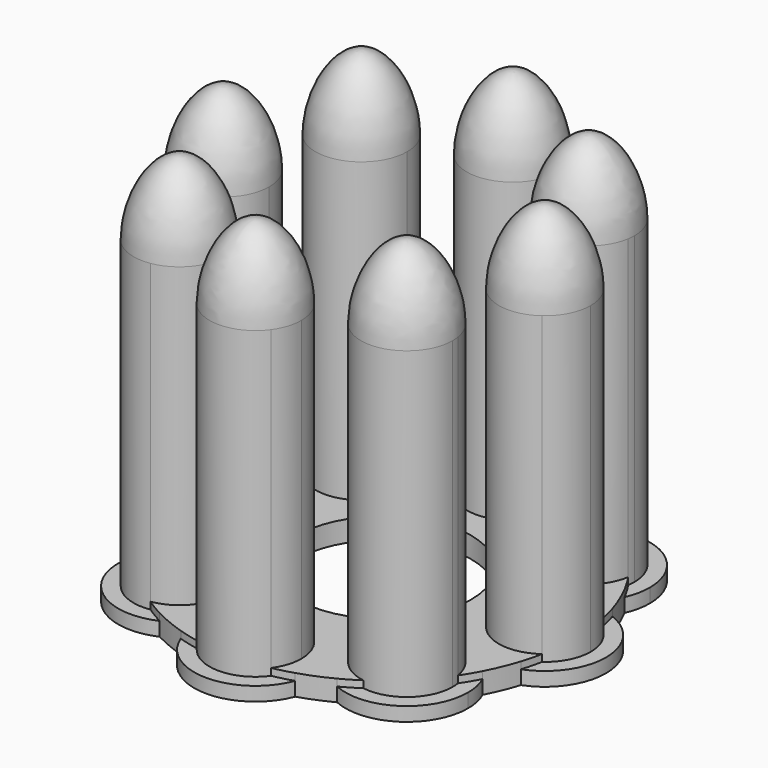
from build123d import *

# Parameters (mm, degrees)
F0_R            = 7.9375
F1_DEPTH        = 0.635
F2_DEPTH        = 1.27
F3_DEPTH        = 27.813
F5_COPIES_COUNT = 8


# Not quite as in the source:
# - a pattern or mirror of a feature is missing from the dataset's text; its kind, count and spacing are read off the source's solid


with BuildPart() as f1:
    # F0 (on Top) → F1 (new body)
    with BuildSketch(Plane.XY):
        with BuildLine():
            ThreePointArc((-5.219470135, 16.6642142857), (-1.0147277679, 9.1734047727), (5.588, 14.6685))
            ThreePointArc((5.588, 14.6685), (5.4950952273, 15.6832277679), (5.219470135, 16.6642142857))
            ThreePointArc((5.219470135, 16.6642142857), (4.3120566918, 16.9217337568), (3.3920620288, 17.1298809524))
            ThreePointArc((3.3920620288, 17.1298809524), (3.986264728, 15.96239896), (4.191, 14.6685))
            ThreePointArc((4.191, 14.6685), (-1.29389896, 10.682235272), (-3.3920620288, 17.1298809524))
            ThreePointArc((-3.3920620288, 17.1298809524), (-4.3120566918, 16.9217337568), (-5.219470135, 16.6642142857))
        make_face()
        with BuildLine():
            ThreePointArc((9.7141049196, 14.5112050451), (8.9163881613, 15.0145572165), (8.0926561979, 15.4741016512))
            ThreePointArc((8.0926561979, 15.4741016512), (6.4208831266, 6.4208831266), (15.4741016512, 8.0926561979))
            ThreePointArc((15.4741016512, 8.0926561979), (15.0145572165, 8.9163881613), (14.5112050451, 9.7141049196))
            ThreePointArc((14.5112050451, 9.7141049196), (7.4087112999, 7.4087112999), (9.7141049196, 14.5112050451))
        make_face()
        with BuildLine():
            ThreePointArc((17.1298809524, 3.3920620288), (16.9217337568, 4.3120566918), (16.6642142857, 5.219470135))
            ThreePointArc((16.6642142857, 5.219470135), (9.0805, 0), (16.6642142857, -5.219470135))
            ThreePointArc((16.6642142857, -5.219470135), (16.9217337568, -4.3120566918), (17.1298809524, -3.3920620288))
            ThreePointArc((17.1298809524, -3.3920620288), (10.4775, 0), (17.1298809524, 3.3920620288))
        make_face()
        with BuildLine():
            ThreePointArc((14.5112050451, -9.7141049196), (15.0145572165, -8.9163881613), (15.4741016512, -8.0926561979))
            ThreePointArc((15.4741016512, -8.0926561979), (6.4208831266, -6.4208831266), (8.0926561979, -15.4741016512))
            ThreePointArc((8.0926561979, -15.4741016512), (8.9163881613, -15.0145572165), (9.7141049196, -14.5112050451))
            ThreePointArc((9.7141049196, -14.5112050451), (7.4087112999, -7.4087112999), (14.5112050451, -9.7141049196))
        make_face()
        with BuildLine():
            ThreePointArc((3.3920620288, -17.1298809524), (4.3120566918, -16.9217337568), (5.219470135, -16.6642142857))
            ThreePointArc((5.219470135, -16.6642142857), (5.4950952273, -15.6832277679), (5.588, -14.6685))
            ThreePointArc((5.588, -14.6685), (-1.0147277679, -9.1734047727), (-5.219470135, -16.6642142857))
            ThreePointArc((-5.219470135, -16.6642142857), (-4.3120566918, -16.9217337568), (-3.3920620288, -17.1298809524))
            ThreePointArc((-3.3920620288, -17.1298809524), (-1.29389896, -10.682235272), (4.191, -14.6685))
            ThreePointArc((4.191, -14.6685), (3.986264728, -15.96239896), (3.3920620288, -17.1298809524))
        make_face()
        with BuildLine():
            ThreePointArc((-4.7841958198, -10.3721958198), (-9.2068001329, -4.907070305), (-15.4741016512, -8.0926561979))
            ThreePointArc((-15.4741016512, -8.0926561979), (-15.0145572165, -8.9163881613), (-14.5112050451, -9.7141049196))
            ThreePointArc((-14.5112050451, -9.7141049196), (-10.0421251177, -6.1942137314), (-6.1811958198, -10.3721958198))
            ThreePointArc((-6.1811958198, -10.3721958198), (-7.1845211216, -13.0930800545), (-9.7141049196, -14.5112050451))
            ThreePointArc((-9.7141049196, -14.5112050451), (-8.9163881613, -15.0145572165), (-8.0926561979, -15.4741016512))
            ThreePointArc((-8.0926561979, -15.4741016512), (-5.6837093153, -13.4125639384), (-4.7841958198, -10.3721958198))
        make_face()
        with BuildLine():
            ThreePointArc((-9.0805, 0), (-11.5004017872, 4.6031399842), (-16.6642142857, 5.219470135))
            ThreePointArc((-16.6642142857, 5.219470135), (-16.9217337568, 4.3120566918), (-17.1298809524, 3.3920620288))
            ThreePointArc((-17.1298809524, 3.3920620288), (-12.764709908, 3.7336395495), (-10.4775, 0))
            ThreePointArc((-10.4775, 0), (-12.764709908, -3.7336395495), (-17.1298809524, -3.3920620288))
            ThreePointArc((-17.1298809524, -3.3920620288), (-16.9217337568, -4.3120566918), (-16.6642142857, -5.219470135))
            ThreePointArc((-16.6642142857, -5.219470135), (-11.5004017872, -4.6031399842), (-9.0805, 0))
        make_face()
        with BuildLine():
            ThreePointArc((-4.7841958198, 10.3721958198), (-5.6837093153, 13.4125639384), (-8.0926561979, 15.4741016512))
            ThreePointArc((-8.0926561979, 15.4741016512), (-8.9163881613, 15.0145572165), (-9.7141049196, 14.5112050451))
            ThreePointArc((-9.7141049196, 14.5112050451), (-7.1845211216, 13.0930800545), (-6.1811958198, 10.3721958198))
            ThreePointArc((-6.1811958198, 10.3721958198), (-10.0421251177, 6.1942137314), (-14.5112050451, 9.7141049196))
            ThreePointArc((-14.5112050451, 9.7141049196), (-15.0145572165, 8.9163881613), (-15.4741016512, 8.0926561979))
            ThreePointArc((-15.4741016512, 8.0926561979), (-9.2068001329, 4.907070305), (-4.7841958198, 10.3721958198))
        make_face()
        with BuildLine():
            ThreePointArc((5.219470135, 16.6642142857), (5.4950952273, 15.6832277679), (5.588, 14.6685))
            ThreePointArc((5.588, 14.6685), (-1.0147277679, 9.1734047727), (-5.219470135, 16.6642142857))
            ThreePointArc((-5.219470135, 16.6642142857), (-6.6826094377, 16.1332463365), (-8.0926561979, 15.4741016512))
            ThreePointArc((-8.0926561979, 15.4741016512), (-5.6837093153, 13.4125639384), (-4.7841958198, 10.3721958198))
            ThreePointArc((-4.7841958198, 10.3721958198), (-9.2068001329, 4.907070305), (-15.4741016512, 8.0926561979))
            ThreePointArc((-15.4741016512, 8.0926561979), (-16.1332463365, 6.6826094377), (-16.6642142857, 5.219470135))
            ThreePointArc((-16.6642142857, 5.219470135), (-11.5004017872, 4.6031399842), (-9.0805, 0))
            ThreePointArc((-9.0805, 0), (-11.5004017872, -4.6031399842), (-16.6642142857, -5.219470135))
            ThreePointArc((-16.6642142857, -5.219470135), (-16.1332463365, -6.6826094377), (-15.4741016512, -8.0926561979))
            ThreePointArc((-15.4741016512, -8.0926561979), (-9.2068001329, -4.907070305), (-4.7841958198, -10.3721958198))
            ThreePointArc((-4.7841958198, -10.3721958198), (-5.6837093153, -13.4125639384), (-8.0926561979, -15.4741016512))
            ThreePointArc((-8.0926561979, -15.4741016512), (-6.6826094377, -16.1332463365), (-5.219470135, -16.6642142857))
            ThreePointArc((-5.219470135, -16.6642142857), (-1.0147277679, -9.1734047727), (5.588, -14.6685))
            ThreePointArc((5.588, -14.6685), (5.4950952273, -15.6832277679), (5.219470135, -16.6642142857))
            ThreePointArc((5.219470135, -16.6642142857), (6.6826094377, -16.1332463365), (8.0926561979, -15.4741016512))
            ThreePointArc((8.0926561979, -15.4741016512), (6.4208831266, -6.4208831266), (15.4741016512, -8.0926561979))
            ThreePointArc((15.4741016512, -8.0926561979), (16.1332463365, -6.6826094377), (16.6642142857, -5.219470135))
            ThreePointArc((16.6642142857, -5.219470135), (9.0805, 0), (16.6642142857, 5.219470135))
            ThreePointArc((16.6642142857, 5.219470135), (16.1332463365, 6.6826094377), (15.4741016512, 8.0926561979))
            ThreePointArc((15.4741016512, 8.0926561979), (6.4208831266, 6.4208831266), (8.0926561979, 15.4741016512))
            ThreePointArc((8.0926561979, 15.4741016512), (6.6826094377, 16.1332463365), (5.219470135, 16.6642142857))
        make_face()
        Circle(F0_R, mode=Mode.SUBTRACT)
    extrude(amount=F1_DEPTH)

    # F0 (on Top) → F2 (join)
    with BuildSketch(Plane.XY):
        with BuildLine():
            ThreePointArc((-5.219470135, 16.6642142857), (-1.0147277679, 9.1734047727), (5.588, 14.6685))
            ThreePointArc((5.588, 14.6685), (5.4950952273, 15.6832277679), (5.219470135, 16.6642142857))
            ThreePointArc((5.219470135, 16.6642142857), (4.3120566918, 16.9217337568), (3.3920620288, 17.1298809524))
            ThreePointArc((3.3920620288, 17.1298809524), (3.986264728, 15.96239896), (4.191, 14.6685))
            ThreePointArc((4.191, 14.6685), (-1.29389896, 10.682235272), (-3.3920620288, 17.1298809524))
            ThreePointArc((-3.3920620288, 17.1298809524), (-4.3120566918, 16.9217337568), (-5.219470135, 16.6642142857))
        make_face()
        with BuildLine():
            ThreePointArc((5.219470135, 16.6642142857), (5.4950952273, 15.6832277679), (5.588, 14.6685))
            ThreePointArc((5.588, 14.6685), (-1.0147277679, 9.1734047727), (-5.219470135, 16.6642142857))
            ThreePointArc((-5.219470135, 16.6642142857), (-6.6826094377, 16.1332463365), (-8.0926561979, 15.4741016512))
            ThreePointArc((-8.0926561979, 15.4741016512), (-5.6837093153, 13.4125639384), (-4.7841958198, 10.3721958198))
            ThreePointArc((-4.7841958198, 10.3721958198), (-9.2068001329, 4.907070305), (-15.4741016512, 8.0926561979))
            ThreePointArc((-15.4741016512, 8.0926561979), (-16.1332463365, 6.6826094377), (-16.6642142857, 5.219470135))
            ThreePointArc((-16.6642142857, 5.219470135), (-11.5004017872, 4.6031399842), (-9.0805, 0))
            ThreePointArc((-9.0805, 0), (-11.5004017872, -4.6031399842), (-16.6642142857, -5.219470135))
            ThreePointArc((-16.6642142857, -5.219470135), (-16.1332463365, -6.6826094377), (-15.4741016512, -8.0926561979))
            ThreePointArc((-15.4741016512, -8.0926561979), (-9.2068001329, -4.907070305), (-4.7841958198, -10.3721958198))
            ThreePointArc((-4.7841958198, -10.3721958198), (-5.6837093153, -13.4125639384), (-8.0926561979, -15.4741016512))
            ThreePointArc((-8.0926561979, -15.4741016512), (-6.6826094377, -16.1332463365), (-5.219470135, -16.6642142857))
            ThreePointArc((-5.219470135, -16.6642142857), (-1.0147277679, -9.1734047727), (5.588, -14.6685))
            ThreePointArc((5.588, -14.6685), (5.4950952273, -15.6832277679), (5.219470135, -16.6642142857))
            ThreePointArc((5.219470135, -16.6642142857), (6.6826094377, -16.1332463365), (8.0926561979, -15.4741016512))
            ThreePointArc((8.0926561979, -15.4741016512), (6.4208831266, -6.4208831266), (15.4741016512, -8.0926561979))
            ThreePointArc((15.4741016512, -8.0926561979), (16.1332463365, -6.6826094377), (16.6642142857, -5.219470135))
            ThreePointArc((16.6642142857, -5.219470135), (9.0805, 0), (16.6642142857, 5.219470135))
            ThreePointArc((16.6642142857, 5.219470135), (16.1332463365, 6.6826094377), (15.4741016512, 8.0926561979))
            ThreePointArc((15.4741016512, 8.0926561979), (6.4208831266, 6.4208831266), (8.0926561979, 15.4741016512))
            ThreePointArc((8.0926561979, 15.4741016512), (6.6826094377, 16.1332463365), (5.219470135, 16.6642142857))
        make_face()
        Circle(F0_R, mode=Mode.SUBTRACT)
        with BuildLine():
            ThreePointArc((3.3920620288, 17.1298809524), (4.3120566918, 16.9217337568), (5.219470135, 16.6642142857))
            ThreePointArc((5.219470135, 16.6642142857), (0, 20.2565), (-5.219470135, 16.6642142857))
            ThreePointArc((-5.219470135, 16.6642142857), (-4.3120566918, 16.9217337568), (-3.3920620288, 17.1298809524))
            ThreePointArc((-3.3920620288, 17.1298809524), (0, 18.8595), (3.3920620288, 17.1298809524))
        make_face()
        with BuildLine():
            ThreePointArc((15.9601958198, 10.3721958198), (13.4125639384, 15.0606823244), (8.0926561979, 15.4741016512))
            ThreePointArc((8.0926561979, 15.4741016512), (8.9163881613, 15.0145572165), (9.7141049196, 14.5112050451))
            ThreePointArc((9.7141049196, 14.5112050451), (13.0930800545, 13.559870518), (14.5631958198, 10.3721958198))
            ThreePointArc((14.5631958198, 10.3721958198), (14.5501779083, 10.0421251177), (14.5112050451, 9.7141049196))
            ThreePointArc((14.5112050451, 9.7141049196), (15.0145572165, 8.9163881613), (15.4741016512, 8.0926561979))
            ThreePointArc((15.4741016512, 8.0926561979), (15.8373213347, 9.2068001329), (15.9601958198, 10.3721958198))
        make_face()
        with BuildLine():
            ThreePointArc((9.7141049196, 14.5112050451), (8.9163881613, 15.0145572165), (8.0926561979, 15.4741016512))
            ThreePointArc((8.0926561979, 15.4741016512), (6.4208831266, 6.4208831266), (15.4741016512, 8.0926561979))
            ThreePointArc((15.4741016512, 8.0926561979), (15.0145572165, 8.9163881613), (14.5112050451, 9.7141049196))
            ThreePointArc((14.5112050451, 9.7141049196), (7.4087112999, 7.4087112999), (9.7141049196, 14.5112050451))
        make_face()
        with BuildLine():
            ThreePointArc((-4.7841958198, 10.3721958198), (-5.6837093153, 13.4125639384), (-8.0926561979, 15.4741016512))
            ThreePointArc((-8.0926561979, 15.4741016512), (-8.9163881613, 15.0145572165), (-9.7141049196, 14.5112050451))
            ThreePointArc((-9.7141049196, 14.5112050451), (-7.1845211216, 13.0930800545), (-6.1811958198, 10.3721958198))
            ThreePointArc((-6.1811958198, 10.3721958198), (-10.0421251177, 6.1942137314), (-14.5112050451, 9.7141049196))
            ThreePointArc((-14.5112050451, 9.7141049196), (-15.0145572165, 8.9163881613), (-15.4741016512, 8.0926561979))
            ThreePointArc((-15.4741016512, 8.0926561979), (-9.2068001329, 4.907070305), (-4.7841958198, 10.3721958198))
        make_face()
        with BuildLine():
            ThreePointArc((-9.7141049196, 14.5112050451), (-8.9163881613, 15.0145572165), (-8.0926561979, 15.4741016512))
            ThreePointArc((-8.0926561979, 15.4741016512), (-14.3235085131, 14.3235085131), (-15.4741016512, 8.0926561979))
            ThreePointArc((-15.4741016512, 8.0926561979), (-15.0145572165, 8.9163881613), (-14.5112050451, 9.7141049196))
            ThreePointArc((-14.5112050451, 9.7141049196), (-13.3356803398, 13.3356803398), (-9.7141049196, 14.5112050451))
        make_face()
        with BuildLine():
            ThreePointArc((20.2565, 0), (19.2716399842, 3.1680982128), (16.6642142857, 5.219470135))
            ThreePointArc((16.6642142857, 5.219470135), (16.9217337568, 4.3120566918), (17.1298809524, 3.3920620288))
            ThreePointArc((17.1298809524, 3.3920620288), (18.4021395495, 1.903790092), (18.8595, 0))
            ThreePointArc((18.8595, 0), (18.4021395495, -1.903790092), (17.1298809524, -3.3920620288))
            ThreePointArc((17.1298809524, -3.3920620288), (16.9217337568, -4.3120566918), (16.6642142857, -5.219470135))
            ThreePointArc((16.6642142857, -5.219470135), (19.2716399842, -3.1680982128), (20.2565, 0))
        make_face()
        with BuildLine():
            ThreePointArc((17.1298809524, 3.3920620288), (16.9217337568, 4.3120566918), (16.6642142857, 5.219470135))
            ThreePointArc((16.6642142857, 5.219470135), (9.0805, 0), (16.6642142857, -5.219470135))
            ThreePointArc((16.6642142857, -5.219470135), (16.9217337568, -4.3120566918), (17.1298809524, -3.3920620288))
            ThreePointArc((17.1298809524, -3.3920620288), (10.4775, 0), (17.1298809524, 3.3920620288))
        make_face()
        with BuildLine():
            ThreePointArc((-9.0805, 0), (-11.5004017872, 4.6031399842), (-16.6642142857, 5.219470135))
            ThreePointArc((-16.6642142857, 5.219470135), (-16.9217337568, 4.3120566918), (-17.1298809524, 3.3920620288))
            ThreePointArc((-17.1298809524, 3.3920620288), (-12.764709908, 3.7336395495), (-10.4775, 0))
            ThreePointArc((-10.4775, 0), (-12.764709908, -3.7336395495), (-17.1298809524, -3.3920620288))
            ThreePointArc((-17.1298809524, -3.3920620288), (-16.9217337568, -4.3120566918), (-16.6642142857, -5.219470135))
            ThreePointArc((-16.6642142857, -5.219470135), (-11.5004017872, -4.6031399842), (-9.0805, 0))
        make_face()
        with BuildLine():
            ThreePointArc((-17.1298809524, 3.3920620288), (-16.9217337568, 4.3120566918), (-16.6642142857, 5.219470135))
            ThreePointArc((-16.6642142857, 5.219470135), (-20.2565, 0), (-16.6642142857, -5.219470135))
            ThreePointArc((-16.6642142857, -5.219470135), (-16.9217337568, -4.3120566918), (-17.1298809524, -3.3920620288))
            ThreePointArc((-17.1298809524, -3.3920620288), (-18.8595, 0), (-17.1298809524, 3.3920620288))
        make_face()
        with BuildLine():
            ThreePointArc((15.9601958198, -10.3721958198), (15.8373213347, -9.2068001329), (15.4741016512, -8.0926561979))
            ThreePointArc((15.4741016512, -8.0926561979), (15.0145572165, -8.9163881613), (14.5112050451, -9.7141049196))
            ThreePointArc((14.5112050451, -9.7141049196), (14.5501779083, -10.0421251177), (14.5631958198, -10.3721958198))
            ThreePointArc((14.5631958198, -10.3721958198), (13.0930800545, -13.559870518), (9.7141049196, -14.5112050451))
            ThreePointArc((9.7141049196, -14.5112050451), (8.9163881613, -15.0145572165), (8.0926561979, -15.4741016512))
            ThreePointArc((8.0926561979, -15.4741016512), (13.4125639384, -15.0606823244), (15.9601958198, -10.3721958198))
        make_face()
        with BuildLine():
            ThreePointArc((14.5112050451, -9.7141049196), (15.0145572165, -8.9163881613), (15.4741016512, -8.0926561979))
            ThreePointArc((15.4741016512, -8.0926561979), (6.4208831266, -6.4208831266), (8.0926561979, -15.4741016512))
            ThreePointArc((8.0926561979, -15.4741016512), (8.9163881613, -15.0145572165), (9.7141049196, -14.5112050451))
            ThreePointArc((9.7141049196, -14.5112050451), (7.4087112999, -7.4087112999), (14.5112050451, -9.7141049196))
        make_face()
        with BuildLine():
            ThreePointArc((-4.7841958198, -10.3721958198), (-9.2068001329, -4.907070305), (-15.4741016512, -8.0926561979))
            ThreePointArc((-15.4741016512, -8.0926561979), (-15.0145572165, -8.9163881613), (-14.5112050451, -9.7141049196))
            ThreePointArc((-14.5112050451, -9.7141049196), (-10.0421251177, -6.1942137314), (-6.1811958198, -10.3721958198))
            ThreePointArc((-6.1811958198, -10.3721958198), (-7.1845211216, -13.0930800545), (-9.7141049196, -14.5112050451))
            ThreePointArc((-9.7141049196, -14.5112050451), (-8.9163881613, -15.0145572165), (-8.0926561979, -15.4741016512))
            ThreePointArc((-8.0926561979, -15.4741016512), (-5.6837093153, -13.4125639384), (-4.7841958198, -10.3721958198))
        make_face()
        with BuildLine():
            ThreePointArc((-14.5112050451, -9.7141049196), (-15.0145572165, -8.9163881613), (-15.4741016512, -8.0926561979))
            ThreePointArc((-15.4741016512, -8.0926561979), (-14.3235085131, -14.3235085131), (-8.0926561979, -15.4741016512))
            ThreePointArc((-8.0926561979, -15.4741016512), (-8.9163881613, -15.0145572165), (-9.7141049196, -14.5112050451))
            ThreePointArc((-9.7141049196, -14.5112050451), (-13.3356803398, -13.3356803398), (-14.5112050451, -9.7141049196))
        make_face()
        with BuildLine():
            ThreePointArc((-5.219470135, -16.6642142857), (0, -20.2565), (5.219470135, -16.6642142857))
            ThreePointArc((5.219470135, -16.6642142857), (4.3120566918, -16.9217337568), (3.3920620288, -17.1298809524))
            ThreePointArc((3.3920620288, -17.1298809524), (0, -18.8595), (-3.3920620288, -17.1298809524))
            ThreePointArc((-3.3920620288, -17.1298809524), (-4.3120566918, -16.9217337568), (-5.219470135, -16.6642142857))
        make_face()
        with BuildLine():
            ThreePointArc((3.3920620288, -17.1298809524), (4.3120566918, -16.9217337568), (5.219470135, -16.6642142857))
            ThreePointArc((5.219470135, -16.6642142857), (5.4950952273, -15.6832277679), (5.588, -14.6685))
            ThreePointArc((5.588, -14.6685), (-1.0147277679, -9.1734047727), (-5.219470135, -16.6642142857))
            ThreePointArc((-5.219470135, -16.6642142857), (-4.3120566918, -16.9217337568), (-3.3920620288, -17.1298809524))
            ThreePointArc((-3.3920620288, -17.1298809524), (-1.29389896, -10.682235272), (4.191, -14.6685))
            ThreePointArc((4.191, -14.6685), (3.986264728, -15.96239896), (3.3920620288, -17.1298809524))
        make_face()
        with BuildLine():
            ThreePointArc((-3.3920620288, -17.1298809524), (0, -18.8595), (3.3920620288, -17.1298809524))
            ThreePointArc((3.3920620288, -17.1298809524), (0, -17.4625), (-3.3920620288, -17.1298809524))
        make_face()
        with BuildLine():
            ThreePointArc((-3.3920620288, -17.1298809524), (0, -17.4625), (3.3920620288, -17.1298809524))
            ThreePointArc((3.3920620288, -17.1298809524), (3.986264728, -15.96239896), (4.191, -14.6685))
            ThreePointArc((4.191, -14.6685), (-1.29389896, -10.682235272), (-3.3920620288, -17.1298809524))
        make_face()
        with BuildLine():
            ThreePointArc((9.7141049196, -14.5112050451), (12.3478521665, -12.3478521665), (14.5112050451, -9.7141049196))
            ThreePointArc((14.5112050451, -9.7141049196), (7.4087112999, -7.4087112999), (9.7141049196, -14.5112050451))
        make_face()
        with BuildLine():
            ThreePointArc((14.5631958198, -10.3721958198), (14.5501779083, -10.0421251177), (14.5112050451, -9.7141049196))
            ThreePointArc((14.5112050451, -9.7141049196), (12.3478521665, -12.3478521665), (9.7141049196, -14.5112050451))
            ThreePointArc((9.7141049196, -14.5112050451), (13.0930800545, -13.559870518), (14.5631958198, -10.3721958198))
        make_face()
        with BuildLine():
            ThreePointArc((18.8595, 0), (18.4021395495, 1.903790092), (17.1298809524, 3.3920620288))
            ThreePointArc((17.1298809524, 3.3920620288), (17.3791463021, 1.7041655024), (17.4625, 0))
            ThreePointArc((17.4625, 0), (17.3791463021, -1.7041655024), (17.1298809524, -3.3920620288))
            ThreePointArc((17.1298809524, -3.3920620288), (18.4021395495, -1.903790092), (18.8595, 0))
        make_face()
        with BuildLine():
            ThreePointArc((17.4625, 0), (17.3791463021, 1.7041655024), (17.1298809524, 3.3920620288))
            ThreePointArc((17.1298809524, 3.3920620288), (10.4775, 0), (17.1298809524, -3.3920620288))
            ThreePointArc((17.1298809524, -3.3920620288), (17.3791463021, -1.7041655024), (17.4625, 0))
        make_face()
        with BuildLine():
            ThreePointArc((14.5112050451, 9.7141049196), (12.3478521665, 12.3478521665), (9.7141049196, 14.5112050451))
            ThreePointArc((9.7141049196, 14.5112050451), (7.4087112999, 7.4087112999), (14.5112050451, 9.7141049196))
        make_face()
        with BuildLine():
            ThreePointArc((14.5631958198, 10.3721958198), (13.0930800545, 13.559870518), (9.7141049196, 14.5112050451))
            ThreePointArc((9.7141049196, 14.5112050451), (12.3478521665, 12.3478521665), (14.5112050451, 9.7141049196))
            ThreePointArc((14.5112050451, 9.7141049196), (14.5501779083, 10.0421251177), (14.5631958198, 10.3721958198))
        make_face()
        with BuildLine():
            ThreePointArc((-6.1811958198, 10.3721958198), (-7.1845211216, 13.0930800545), (-9.7141049196, 14.5112050451))
            ThreePointArc((-9.7141049196, 14.5112050451), (-12.3478521665, 12.3478521665), (-14.5112050451, 9.7141049196))
            ThreePointArc((-14.5112050451, 9.7141049196), (-10.0421251177, 6.1942137314), (-6.1811958198, 10.3721958198))
        make_face()
        with BuildLine():
            ThreePointArc((-14.5112050451, 9.7141049196), (-12.3478521665, 12.3478521665), (-9.7141049196, 14.5112050451))
            ThreePointArc((-9.7141049196, 14.5112050451), (-13.3356803398, 13.3356803398), (-14.5112050451, 9.7141049196))
        make_face()
        with BuildLine():
            ThreePointArc((-10.4775, 0), (-12.764709908, 3.7336395495), (-17.1298809524, 3.3920620288))
            ThreePointArc((-17.1298809524, 3.3920620288), (-17.4625, 0), (-17.1298809524, -3.3920620288))
            ThreePointArc((-17.1298809524, -3.3920620288), (-12.764709908, -3.7336395495), (-10.4775, 0))
        make_face()
        with BuildLine():
            ThreePointArc((4.191, 14.6685), (3.986264728, 15.96239896), (3.3920620288, 17.1298809524))
            ThreePointArc((3.3920620288, 17.1298809524), (0, 17.4625), (-3.3920620288, 17.1298809524))
            ThreePointArc((-3.3920620288, 17.1298809524), (-1.29389896, 10.682235272), (4.191, 14.6685))
        make_face()
        with BuildLine():
            ThreePointArc((-3.3920620288, 17.1298809524), (0, 17.4625), (3.3920620288, 17.1298809524))
            ThreePointArc((3.3920620288, 17.1298809524), (0, 18.8595), (-3.3920620288, 17.1298809524))
        make_face()
        with BuildLine():
            ThreePointArc((-9.7141049196, -14.5112050451), (-12.3478521665, -12.3478521665), (-14.5112050451, -9.7141049196))
            ThreePointArc((-14.5112050451, -9.7141049196), (-13.3356803398, -13.3356803398), (-9.7141049196, -14.5112050451))
        make_face()
        with BuildLine():
            ThreePointArc((-6.1811958198, -10.3721958198), (-10.0421251177, -6.1942137314), (-14.5112050451, -9.7141049196))
            ThreePointArc((-14.5112050451, -9.7141049196), (-12.3478521665, -12.3478521665), (-9.7141049196, -14.5112050451))
            ThreePointArc((-9.7141049196, -14.5112050451), (-7.1845211216, -13.0930800545), (-6.1811958198, -10.3721958198))
        make_face()
        with BuildLine():
            ThreePointArc((-17.1298809524, -3.3920620288), (-17.4625, 0), (-17.1298809524, 3.3920620288))
            ThreePointArc((-17.1298809524, 3.3920620288), (-18.8595, 0), (-17.1298809524, -3.3920620288))
        make_face()
    extrude(amount=-F2_DEPTH)

    # F0 (on Top) → F3 (join)
    with BuildSketch(Plane.XY):
        with BuildLine():
            ThreePointArc((9.7141049196, -14.5112050451), (12.3478521665, -12.3478521665), (14.5112050451, -9.7141049196))
            ThreePointArc((14.5112050451, -9.7141049196), (7.4087112999, -7.4087112999), (9.7141049196, -14.5112050451))
        make_face()
        with BuildLine():
            ThreePointArc((14.5631958198, -10.3721958198), (14.5501779083, -10.0421251177), (14.5112050451, -9.7141049196))
            ThreePointArc((14.5112050451, -9.7141049196), (12.3478521665, -12.3478521665), (9.7141049196, -14.5112050451))
            ThreePointArc((9.7141049196, -14.5112050451), (13.0930800545, -13.559870518), (14.5631958198, -10.3721958198))
        make_face()
        with BuildLine():
            ThreePointArc((-3.3920620288, -17.1298809524), (0, -18.8595), (3.3920620288, -17.1298809524))
            ThreePointArc((3.3920620288, -17.1298809524), (0, -17.4625), (-3.3920620288, -17.1298809524))
        make_face()
        with BuildLine():
            ThreePointArc((-3.3920620288, -17.1298809524), (0, -17.4625), (3.3920620288, -17.1298809524))
            ThreePointArc((3.3920620288, -17.1298809524), (3.986264728, -15.96239896), (4.191, -14.6685))
            ThreePointArc((4.191, -14.6685), (-1.29389896, -10.682235272), (-3.3920620288, -17.1298809524))
        make_face()
        with BuildLine():
            ThreePointArc((-6.1811958198, -10.3721958198), (-10.0421251177, -6.1942137314), (-14.5112050451, -9.7141049196))
            ThreePointArc((-14.5112050451, -9.7141049196), (-12.3478521665, -12.3478521665), (-9.7141049196, -14.5112050451))
            ThreePointArc((-9.7141049196, -14.5112050451), (-7.1845211216, -13.0930800545), (-6.1811958198, -10.3721958198))
        make_face()
        with BuildLine():
            ThreePointArc((-9.7141049196, -14.5112050451), (-12.3478521665, -12.3478521665), (-14.5112050451, -9.7141049196))
            ThreePointArc((-14.5112050451, -9.7141049196), (-13.3356803398, -13.3356803398), (-9.7141049196, -14.5112050451))
        make_face()
        with BuildLine():
            ThreePointArc((-10.4775, 0), (-12.764709908, 3.7336395495), (-17.1298809524, 3.3920620288))
            ThreePointArc((-17.1298809524, 3.3920620288), (-17.4625, 0), (-17.1298809524, -3.3920620288))
            ThreePointArc((-17.1298809524, -3.3920620288), (-12.764709908, -3.7336395495), (-10.4775, 0))
        make_face()
        with BuildLine():
            ThreePointArc((-17.1298809524, -3.3920620288), (-17.4625, 0), (-17.1298809524, 3.3920620288))
            ThreePointArc((-17.1298809524, 3.3920620288), (-18.8595, 0), (-17.1298809524, -3.3920620288))
        make_face()
        with BuildLine():
            ThreePointArc((-6.1811958198, 10.3721958198), (-7.1845211216, 13.0930800545), (-9.7141049196, 14.5112050451))
            ThreePointArc((-9.7141049196, 14.5112050451), (-12.3478521665, 12.3478521665), (-14.5112050451, 9.7141049196))
            ThreePointArc((-14.5112050451, 9.7141049196), (-10.0421251177, 6.1942137314), (-6.1811958198, 10.3721958198))
        make_face()
        with BuildLine():
            ThreePointArc((-14.5112050451, 9.7141049196), (-12.3478521665, 12.3478521665), (-9.7141049196, 14.5112050451))
            ThreePointArc((-9.7141049196, 14.5112050451), (-13.3356803398, 13.3356803398), (-14.5112050451, 9.7141049196))
        make_face()
        with BuildLine():
            ThreePointArc((4.191, 14.6685), (3.986264728, 15.96239896), (3.3920620288, 17.1298809524))
            ThreePointArc((3.3920620288, 17.1298809524), (0, 17.4625), (-3.3920620288, 17.1298809524))
            ThreePointArc((-3.3920620288, 17.1298809524), (-1.29389896, 10.682235272), (4.191, 14.6685))
        make_face()
        with BuildLine():
            ThreePointArc((-3.3920620288, 17.1298809524), (0, 17.4625), (3.3920620288, 17.1298809524))
            ThreePointArc((3.3920620288, 17.1298809524), (0, 18.8595), (-3.3920620288, 17.1298809524))
        make_face()
        with BuildLine():
            ThreePointArc((14.5112050451, 9.7141049196), (12.3478521665, 12.3478521665), (9.7141049196, 14.5112050451))
            ThreePointArc((9.7141049196, 14.5112050451), (7.4087112999, 7.4087112999), (14.5112050451, 9.7141049196))
        make_face()
        with BuildLine():
            ThreePointArc((14.5631958198, 10.3721958198), (13.0930800545, 13.559870518), (9.7141049196, 14.5112050451))
            ThreePointArc((9.7141049196, 14.5112050451), (12.3478521665, 12.3478521665), (14.5112050451, 9.7141049196))
            ThreePointArc((14.5112050451, 9.7141049196), (14.5501779083, 10.0421251177), (14.5631958198, 10.3721958198))
        make_face()
        with BuildLine():
            ThreePointArc((17.4625, 0), (17.3791463021, 1.7041655024), (17.1298809524, 3.3920620288))
            ThreePointArc((17.1298809524, 3.3920620288), (10.4775, 0), (17.1298809524, -3.3920620288))
            ThreePointArc((17.1298809524, -3.3920620288), (17.3791463021, -1.7041655024), (17.4625, 0))
        make_face()
        with BuildLine():
            ThreePointArc((18.8595, 0), (18.4021395495, 1.903790092), (17.1298809524, 3.3920620288))
            ThreePointArc((17.1298809524, 3.3920620288), (17.3791463021, 1.7041655024), (17.4625, 0))
            ThreePointArc((17.4625, 0), (17.3791463021, -1.7041655024), (17.1298809524, -3.3920620288))
            ThreePointArc((17.1298809524, -3.3920620288), (18.4021395495, -1.903790092), (18.8595, 0))
        make_face()
    extrude(amount=F3_DEPTH)

    # F4 (on Right) → F5 (revolve)
    with BuildSketch(Plane.YZ):
        with BuildLine():
            Line((14.6685, 34.671), (14.6685, 27.813))
            Line((14.6685, 27.813), (18.8595, 27.813))
            add(Edge.make_bspline(
                [(14.6685, 34.671), (16.764, 34.671), (18.8595, 31.242), (18.8595, 27.813)],
                knots=[0, 0, 0, 0, 8.0372038048, 8.0372038048, 8.0372038048, 8.0372038048], degree=3))
        make_face()
    f5 = revolve(axis=Axis((0, 14.6685, 31.242), (0, 0, 1)))

    # F5_copies: F5 ×8 about axis
    f5_copies_axis = Axis((0, 0, 0), (0, 0, 1))
    for i in range(1, F5_COPIES_COUNT):
        add(f5.rotate(f5_copies_axis, i * 360 / F5_COPIES_COUNT))


solid = f1.part
